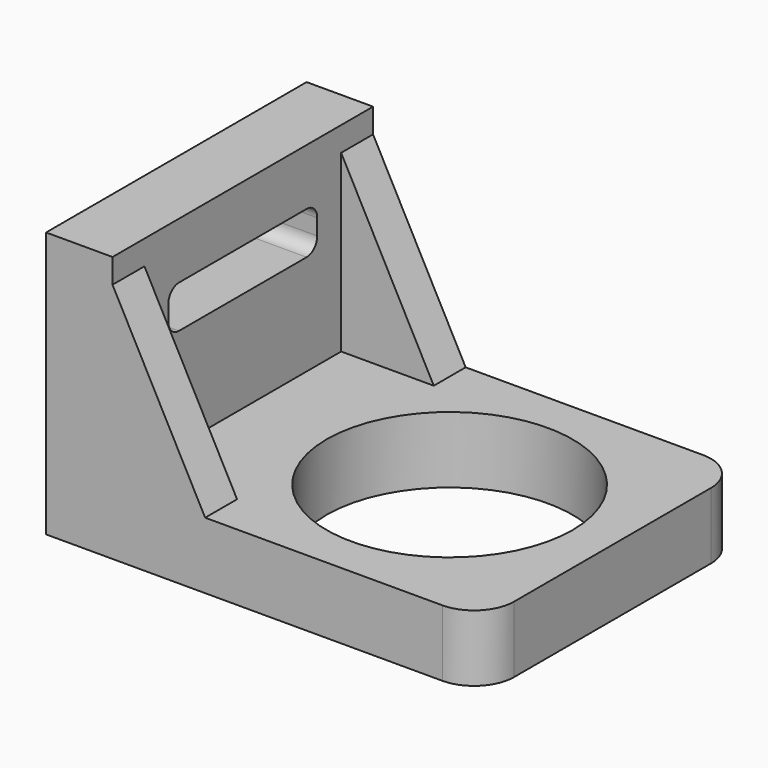
from build123d import *

# Parameters (mm, degrees)
F0_W     = 32.809374243
F0_H     = 24.5
F0_R     = 9.25
F1_DEPTH = 5
F2_W     = 5
F2_H     = 24.5
F3_DEPTH = 15
F5_DEPTH = 3
F6_W     = 14
F6_H     = 3.2
F7_DEPTH = 25
F8_R     = 1
F9_R     = 3


# Not quite as in the source:
# - a pattern or mirror of a feature is missing from the dataset's text; its kind, count and spacing are read off the source's solid


with BuildPart() as f1:
    # F0 (on Top) → F1 (new body)
    with BuildSketch(Plane.XY):
        with Locations((-4.1546871215, 0)):
            Rectangle(F0_W, F0_H)
        Circle(F0_R, mode=Mode.SUBTRACT)
    extrude(amount=F1_DEPTH)

    # F2 (on face) → F3 (join)
    with BuildSketch(Plane.XY.offset(5)):
        with Locations((-18.059374243, 0)):
            Rectangle(F2_W, F2_H)
    extrude(amount=F3_DEPTH)

    # F4 (on face) → F5 (join)
    with BuildSketch(Plane.XZ.offset(12.25)):
        Polygon((-8.5921417922, 5), (-15.559374243, 18.1631296873), (-15.559374243, 5), align=None)
    f5 = extrude(amount=-F5_DEPTH)

    # F5_copies: F5 across plane
    add(f5.mirror(Plane.ZX))

    # F6 (on face) → F7 (cut)
    with BuildSketch(Plane.YZ.offset(-15.559374243)):
        with Locations((0, 14.1660655677)):
            Rectangle(F6_W, F6_H)
    extrude(amount=-F7_DEPTH, mode=Mode.SUBTRACT)

    # F8
    f8_edges = [f1.edges().sort_by_distance(p)[0] for p in [
        (-18.059374, 7, 12.566066),
        (-18.059374, 7, 15.766066),
        (-18.059374, -7, 12.566066),
        (-18.059374, -7, 15.766066),
    ]]
    fillet(f8_edges, radius=F8_R)

    # F9
    f9_edges = [f1.edges().sort_by_distance(p)[0] for p in [
        (12.25, -12.25, 2.5),
        (12.25, 12.25, 2.5),
    ]]
    fillet(f9_edges, radius=F9_R)


solid = f1.part
